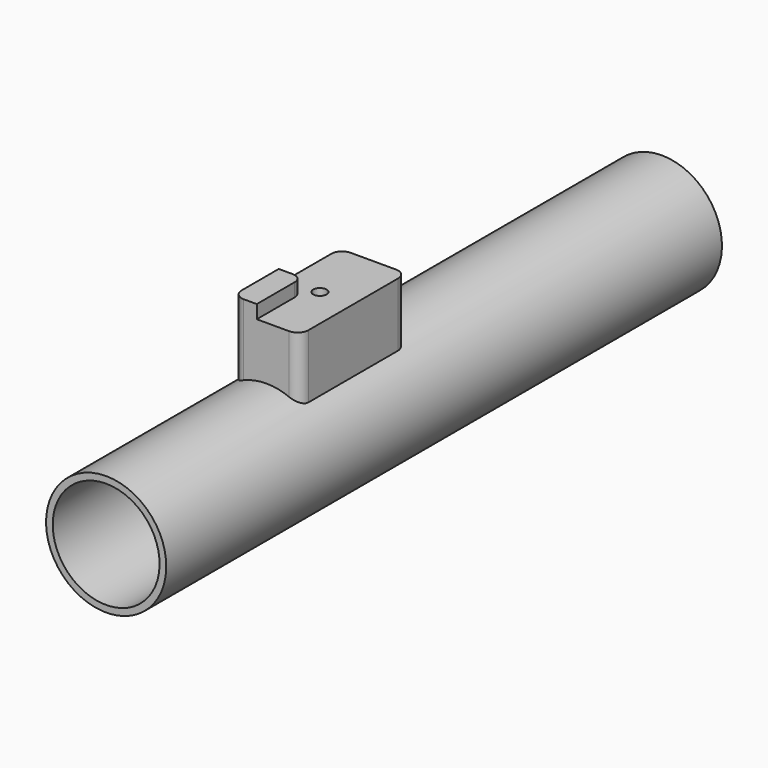
from build123d import *

# Parameters (mm, degrees)
F2_DEPTH = 12.5
F4_DEPTH = 50
F6_D     = 5
F6_DEPTH = 50
F6_TIP   = 1.5021515476
F7_W     = 8.875
F7_H     = 21.375
F8_DEPTH = 5
F9_R     = 3.625
F10_R    = 4


# Not quite as in the source:
# - a feature names something its author has since deleted; it is built from what else it names


with BuildPart() as f1:
    # F0 (on Right) → F1 (revolve)
    with BuildSketch(Plane.YZ):
        Polygon((-25, 22.5), (-100, 22.5), (-100, 20), (0, 20), (100, 20), (160, 20), (160, 22.5), (100, 22.5), (25, 22.5), (0, 22.5), align=None)
    revolve(axis=Axis((0, 2.0652181371, 0), (0, 1, 0)))

    # F0 (on Right) → F2 (join, symmetric)
    with BuildSketch(Plane.YZ):
        Polygon((-25, 42.5), (-25, 22.5), (0, 22.5), (25, 22.5), (25, 42.5), (0, 42.5), align=None)
    extrude(amount=F2_DEPTH, both=True)

    # F3 (on face) → F4 (join)
    with BuildSketch(Plane(origin=(0, 25, 0), x_dir=(-1, 0, 0), z_dir=(0, 1, 0))):
        Polygon((0, 22.5), (-12.5, 22.5), (-12.5, 18.6568256468), align=None)
        Polygon((12.5, 22.5), (0, 22.5), (12.5, 18.6568256468), align=None)
    extrude(amount=-F4_DEPTH)

    # F6
    with Locations(Plane.XY.offset(42.5)):
        with Locations((0, 0)):
            Hole(F6_D / 2, depth=F6_DEPTH)
            with Locations((0, 0, -(F6_DEPTH + F6_TIP / 2))):  # 118° drill point
                Cone(0, F6_D / 2, F6_TIP, mode=Mode.SUBTRACT)

    # F7 (on face) → F8 (join)
    with BuildSketch(Plane.XY.offset(42.5)):
        with Locations((-8.0625, -14.3125)):
            Rectangle(F7_W, F7_H)
    extrude(amount=F8_DEPTH)

    # F9
    f9_edges = [f1.edges().sort_by_distance(p)[0] for p in [
        (-3.625, -3.625, 45),
    ]]
    fillet(f9_edges, radius=F9_R)

    # F10
    f10_edges = [f1.edges().sort_by_distance(p)[0] for p in [
        (12.5, 25, 30.604143),
        (12.5, -25, 30.604143),
        (-12.5, 25, 30.604143),
        (-12.5, -25, 33.104143),
    ]]
    fillet(f10_edges, radius=F10_R)


solid = f1.part
